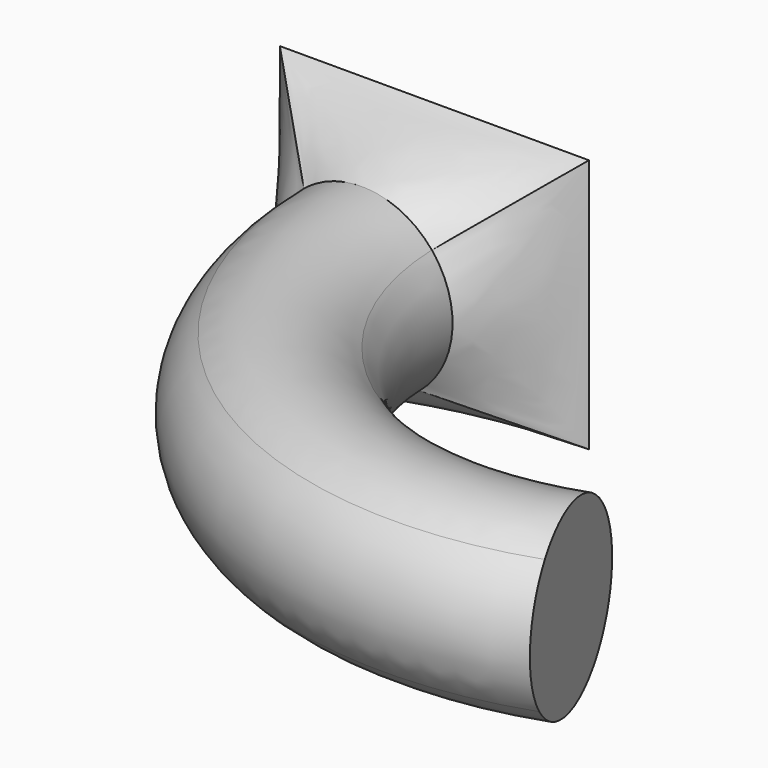
from build123d import *

# Parameters (mm, degrees)
F2_W = 85
F2_H = 70


# Not quite as in the source:
# - the arcs of a loft's sections are written as splines that run evenly, so that the points pair up as in the source's solid


with BuildPart() as f3:
    # F1 (on offset) → F3 section 0
    with BuildSketch(Plane.XZ.offset(25)):
        with BuildLine():
            add(Edge.make_bspline(
                [(19.2982558904, 15.8926813215), (18.2580823303, 17.155749216), (17.0935362371, 18.3163402581), (14.560337759, 20.3880814665), (13.1917480123, 21.2991804049), (10.3030475731, 22.8369111801), (8.7830083094, 23.4635049935), (5.649817047, 24.4081312041), (4.0367425227, 24.7261402436), (0.7794672203, 25.0413604342), (-0.8646530153, 25.0385637908), (-4.1208370946, 24.7122642261), (-5.7328204228, 24.3887693732), (-8.8627799509, 23.4334895626), (-10.3806787565, 22.8017282261), (-13.2641311441, 21.2541790369), (-14.6296134271, 20.3384294505), (-15.8926813215, 19.2982558904)],
                knots=[0, 0, 0, 0, 0.125, 0.125, 0.25, 0.25, 0.375, 0.375, 0.5, 0.5, 0.625, 0.625, 0.75, 0.75, 0.875, 0.875, 1, 1, 1, 1], degree=3))
            add(Edge.make_bspline(
                [(-15.8926813215, 19.2982558904), (-17.155749216, 18.2580823303), (-18.3163402581, 17.0935362371), (-20.3880814665, 14.560337759), (-21.2991804049, 13.1917480123), (-22.8369111801, 10.3030475731), (-23.4635049935, 8.7830083094), (-24.4081312041, 5.649817047), (-24.7261402436, 4.0367425227), (-25.0413604342, 0.7794672203), (-25.0385637908, -0.8646530153), (-24.7122642261, -4.1208370946), (-24.3887693732, -5.7328204228), (-23.4334895626, -8.8627799509), (-22.8017282261, -10.3806787565), (-21.2541790369, -13.2641311441), (-20.3384294505, -14.6296134271), (-19.2982558904, -15.8926813215)],
                knots=[0, 0, 0, 0, 0.125, 0.125, 0.25, 0.25, 0.375, 0.375, 0.5, 0.5, 0.625, 0.625, 0.75, 0.75, 0.875, 0.875, 1, 1, 1, 1], degree=3))
            add(Edge.make_bspline(
                [(-19.2982558904, -15.8926813215), (-18.2580823303, -17.155749216), (-17.0935362371, -18.3163402581), (-14.560337759, -20.3880814665), (-13.1917480123, -21.2991804049), (-10.3030475731, -22.8369111801), (-8.7830083094, -23.4635049935), (-5.649817047, -24.4081312041), (-4.0367425227, -24.7261402436), (-0.7794672203, -25.0413604342), (0.8646530153, -25.0385637908), (4.1208370946, -24.7122642261), (5.7328204228, -24.3887693732), (8.8627799509, -23.4334895626), (10.3806787565, -22.8017282261), (13.2641311441, -21.2541790369), (14.6296134271, -20.3384294505), (15.8926813215, -19.2982558904)],
                knots=[0, 0, 0, 0, 0.125, 0.125, 0.25, 0.25, 0.375, 0.375, 0.5, 0.5, 0.625, 0.625, 0.75, 0.75, 0.875, 0.875, 1, 1, 1, 1], degree=3))
            add(Edge.make_bspline(
                [(15.8926813215, -19.2982558904), (17.155749216, -18.2580823303), (18.3163402581, -17.0935362371), (20.3880814665, -14.560337759), (21.2991804049, -13.1917480123), (22.8369111801, -10.3030475731), (23.4635049935, -8.7830083094), (24.4081312041, -5.649817047), (24.7261402436, -4.0367425227), (25.0413604342, -0.7794672203), (25.0385637908, 0.8646530153), (24.7122642261, 4.1208370946), (24.3887693732, 5.7328204228), (23.4334895626, 8.8627799509), (22.8017282261, 10.3806787565), (21.2541790369, 13.2641311441), (20.3384294505, 14.6296134271), (19.2982558904, 15.8926813215)],
                knots=[0, 0, 0, 0, 0.125, 0.125, 0.25, 0.25, 0.375, 0.375, 0.5, 0.5, 0.625, 0.625, 0.75, 0.75, 0.875, 0.875, 1, 1, 1, 1], degree=3))
        make_face()
    # F2 (on Front) → F3 section 1
    with BuildSketch(Plane.XZ):
        Rectangle(F2_W, F2_H)
    loft(ruled=True)

    # F5: sweep along a path in F4
    with BuildLine(Plane.XY) as f5_path:
        ThreePointArc((0, -25), (41.4671421212, -101.0552801806), (127.3674694821, -112.2384496033))
    # F3_face (on face) → F5 (sweep)
    with BuildSketch(Plane.XZ.offset(25)):
        with BuildLine():
            add(Edge.make_bspline(
                [(19.2982558904, 15.8926813215), (18.2580823303, 17.155749216), (17.0935362371, 18.3163402581), (14.560337759, 20.3880814665), (13.1917480123, 21.2991804049), (10.3030475731, 22.8369111801), (8.7830083094, 23.4635049935), (5.649817047, 24.4081312041), (4.0367425227, 24.7261402436), (0.7794672203, 25.0413604342), (-0.8646530153, 25.0385637908), (-4.1208370946, 24.7122642261), (-5.7328204228, 24.3887693732), (-8.8627799509, 23.4334895626), (-10.3806787565, 22.8017282261), (-13.2641311441, 21.2541790369), (-14.6296134271, 20.3384294505), (-15.8926813215, 19.2982558904)],
                knots=[0, 0, 0, 0, 0.125, 0.125, 0.25, 0.25, 0.375, 0.375, 0.5, 0.5, 0.625, 0.625, 0.75, 0.75, 0.875, 0.875, 1, 1, 1, 1], degree=3))
            add(Edge.make_bspline(
                [(-15.8926813215, 19.2982558904), (-17.155749216, 18.2580823303), (-18.3163402581, 17.0935362371), (-20.3880814665, 14.560337759), (-21.2991804049, 13.1917480123), (-22.8369111801, 10.3030475731), (-23.4635049935, 8.7830083094), (-24.4081312041, 5.649817047), (-24.7261402436, 4.0367425227), (-25.0413604342, 0.7794672203), (-25.0385637908, -0.8646530153), (-24.7122642261, -4.1208370946), (-24.3887693732, -5.7328204228), (-23.4334895626, -8.8627799509), (-22.8017282261, -10.3806787565), (-21.2541790369, -13.2641311441), (-20.3384294505, -14.6296134271), (-19.2982558904, -15.8926813215)],
                knots=[0, 0, 0, 0, 0.125, 0.125, 0.25, 0.25, 0.375, 0.375, 0.5, 0.5, 0.625, 0.625, 0.75, 0.75, 0.875, 0.875, 1, 1, 1, 1], degree=3))
            add(Edge.make_bspline(
                [(-19.2982558904, -15.8926813215), (-18.2580823303, -17.155749216), (-17.0935362371, -18.3163402581), (-14.560337759, -20.3880814665), (-13.1917480123, -21.2991804049), (-10.3030475731, -22.8369111801), (-8.7830083094, -23.4635049935), (-5.649817047, -24.4081312041), (-4.0367425227, -24.7261402436), (-0.7794672203, -25.0413604342), (0.8646530153, -25.0385637908), (4.1208370946, -24.7122642261), (5.7328204228, -24.3887693732), (8.8627799509, -23.4334895626), (10.3806787565, -22.8017282261), (13.2641311441, -21.2541790369), (14.6296134271, -20.3384294505), (15.8926813215, -19.2982558904)],
                knots=[0, 0, 0, 0, 0.125, 0.125, 0.25, 0.25, 0.375, 0.375, 0.5, 0.5, 0.625, 0.625, 0.75, 0.75, 0.875, 0.875, 1, 1, 1, 1], degree=3))
            add(Edge.make_bspline(
                [(15.8926813215, -19.2982558904), (17.155749216, -18.2580823303), (18.3163402581, -17.0935362371), (20.3880814665, -14.560337759), (21.2991804049, -13.1917480123), (22.8369111801, -10.3030475731), (23.4635049935, -8.7830083094), (24.4081312041, -5.649817047), (24.7261402436, -4.0367425227), (25.0413604342, -0.7794672203), (25.0385637908, 0.8646530153), (24.7122642261, 4.1208370946), (24.3887693732, 5.7328204228), (23.4334895626, 8.8627799509), (22.8017282261, 10.3806787565), (21.2541790369, 13.2641311441), (20.3384294505, 14.6296134271), (19.2982558904, 15.8926813215)],
                knots=[0, 0, 0, 0, 0.125, 0.125, 0.25, 0.25, 0.375, 0.375, 0.5, 0.5, 0.625, 0.625, 0.75, 0.75, 0.875, 0.875, 1, 1, 1, 1], degree=3))
        make_face()
    sweep(path=f5_path.line)


solid = f3.part
